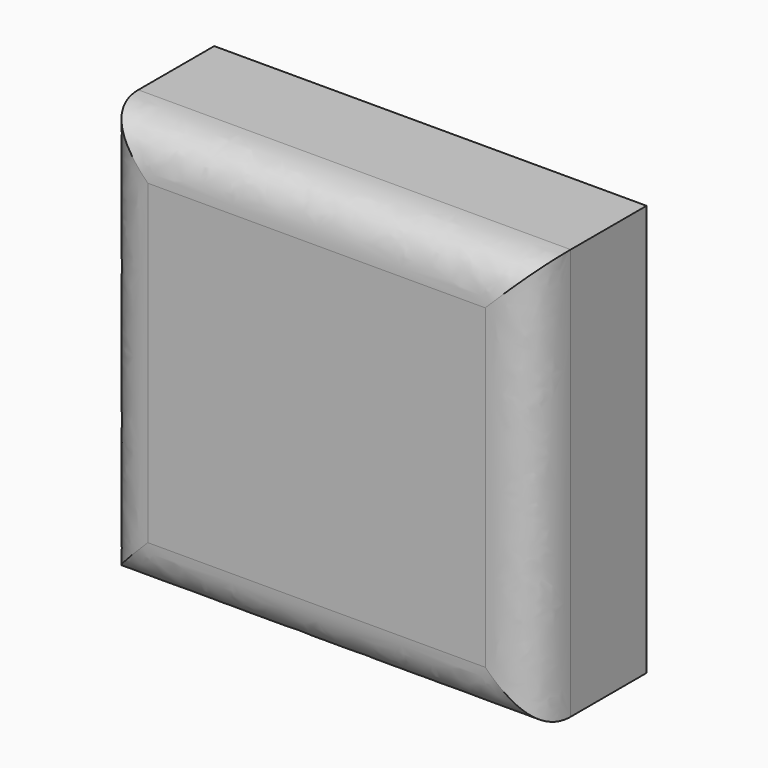
from build123d import *

# Parameters (mm, degrees)
F0_W        = 45.5770306289
F0_H        = 43.3585755527
F1_DEPTH    = 15
F2_T1_DEPTH = 70.5770306289
F2_T3_DEPTH = 68.3585755527


# Not quite as in the source:
# - a fillet or chamfer that OpenCascade refuses, or shapes differently, is made with other operations: its cross-section is extruded or revolved along the edge and cut away or added


with BuildPart() as f1:
    # F0 (on Front) → F1 (new body)
    with BuildSketch(Plane.XZ):
        Rectangle(F0_W, F0_H)
    extrude(amount=F1_DEPTH)

    # F2: fillet of radius 5 on 4 edges, made by hand

    # F2_s2 → F2_t1 (cut)
    with BuildSketch(Plane.YZ.offset(-35.2885153145)):
        with BuildLine():
            add(Edge.make_bspline(
                [(-10, 21.6792877764), (-15, 21.6792877764), (-15, 16.6792877764)],
                knots=[0, 0, 0, 1, 1, 1], degree=2, weights=[1, 1, 1]))
            Line((-15, 16.6792877764), (-15, 21.6792877764))
            Line((-15, 21.6792877764), (-10, 21.6792877764))
        make_face()
        with BuildLine():
            add(Edge.make_bspline(
                [(-10, -21.6792877764), (-15, -21.6792877764), (-15, -16.6792877764)],
                knots=[0, 0, 0, 1, 1, 1], degree=2, weights=[1, 1, 1]))
            Line((-15, -16.6792877764), (-15, -21.6792877764))
            Line((-15, -21.6792877764), (-10, -21.6792877764))
        make_face()
    extrude(amount=F2_T1_DEPTH, mode=Mode.SUBTRACT)

    # F2_s4 → F2_t3 (cut)
    with BuildSketch(Plane.XY.offset(-34.1792877764)):
        with BuildLine():
            add(Edge.make_bspline(
                [(22.7885153145, -10), (22.7885153145, -15), (17.7885153145, -15)],
                knots=[0, 0, 0, 1, 1, 1], degree=2, weights=[1, 1, 1]))
            Line((17.7885153145, -15), (22.7885153145, -15))
            Line((22.7885153145, -15), (22.7885153145, -10))
        make_face()
        with BuildLine():
            add(Edge.make_bspline(
                [(-22.7885153145, -10), (-22.7885153145, -15), (-17.7885153145, -15)],
                knots=[0, 0, 0, 1, 1, 1], degree=2, weights=[1, 1, 1]))
            Line((-17.7885153145, -15), (-22.7885153145, -15))
            Line((-22.7885153145, -15), (-22.7885153145, -10))
        make_face()
    extrude(amount=F2_T3_DEPTH, mode=Mode.SUBTRACT)


solid = f1.part
